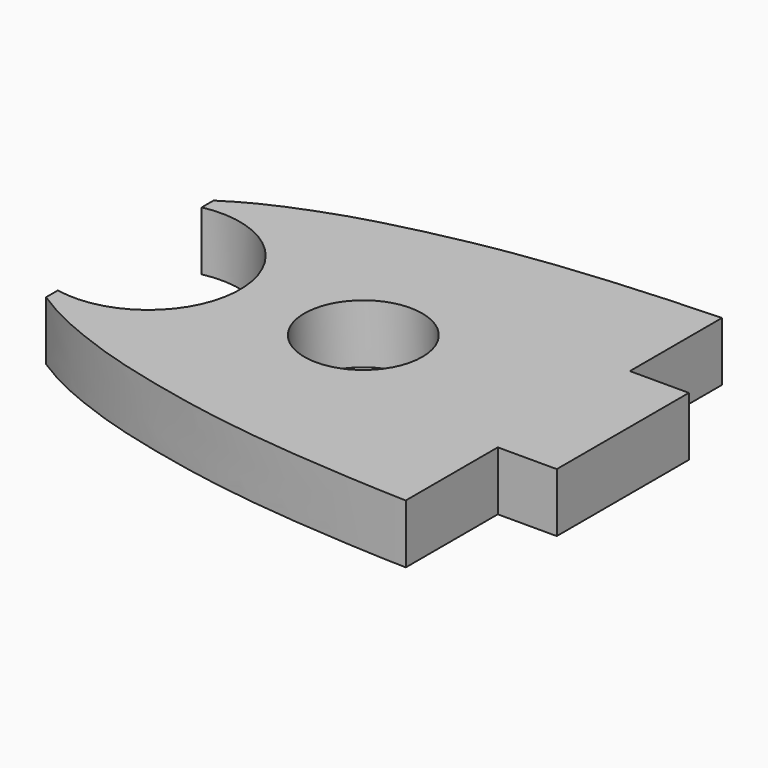
from build123d import *

# Parameters (mm, degrees)
F1_DEPTH      = 3.175
F2_R          = 3.175
F3_DEPTH      = 3.175
F4_W          = 1.27
F4_H          = 6.2519614453
F5_DEPTH      = 25.4
F5_DEPTH_BACK = 25.4


with BuildPart() as f1:
    # F0 (on Top) → F1 (new body)
    with BuildSketch(Plane.XY):
        with BuildLine():
            Line((27.305, 4.445), (27.305, 10.639110318))
            add(Edge.make_bspline(
                [(27.305, 10.639110318), (26.6654543063, 10.6206147569), (24.478766488, 10.5308275824), (20.2410001582, 10.2440182138), (15.3587302448, 9.6192519425), (10.1940451056, 8.4075577542), (7.6509138704, 7.5021601175), (5.5897078561, 6.6511520763), (4.3073818225, 5.8741162544), (3.9357558202, 5.633461687)],
                knots=[0.3056468503, 0.3056468503, 0.3056468503, 0.3056468503, 0.3165359722, 0.343963226, 0.3714836424, 0.3992368185, 0.4191371497, 0.4394264313, 0.4482604373, 0.4482604373, 0.4482604373, 0.4482604373], degree=3))
            Line((3.9357558202, 5.633461687), (3.9357558202, 4.839711687))
            ThreePointArc((3.9357558202, 4.839711687), (9.8679, 0), (3.9357558202, -4.839711687))
            Line((3.9357558202, -4.839711687), (3.9357558202, -5.633461687))
            add(Edge.make_bspline(
                [(3.9357558202, -5.633461687), (4.3073818225, -5.8741162544), (5.5897078561, -6.6511520763), (7.6509138704, -7.5021601175), (10.1940451056, -8.4075577542), (15.3587302448, -9.6192519425), (20.2410001582, -10.2440182138), (24.478766488, -10.5308275824), (26.6654543063, -10.6206147569), (27.305, -10.639110318)],
                knots=[0.5517395627, 0.5517395627, 0.5517395627, 0.5517395627, 0.5605735687, 0.5808628503, 0.6007631815, 0.6285163576, 0.656036774, 0.6834640278, 0.6943531497, 0.6943531497, 0.6943531497, 0.6943531497], degree=3))
            Line((27.305, -10.639110318), (27.305, -4.445))
            Line((27.305, -4.445), (30.48, -4.445))
            Line((30.48, -4.445), (30.48, 4.445))
            Line((30.48, 4.445), (27.305, 4.445))
        make_face()
    extrude(amount=F1_DEPTH)

    # F2 (on face) → F3 (cut, through all)
    with BuildSketch(Plane.XY.offset(3.175)):
        with Locations((16.51, 0)):
            Circle(F2_R)
    extrude(amount=-F3_DEPTH, mode=Mode.SUBTRACT)


with BuildPart() as f1b:
    # F0 (on Top) → F1, piece 2 (new body)
    with BuildSketch(Plane.XY):
        with BuildLine():
            add(Edge.make_bspline(
                [(1.1020531618, 3.1259807227), (0.5678867915, 2.3248543379), (-0.5678867915, 0), (0.5678867915, -2.3248543379), (1.1020531618, -3.1259807227)],
                knots=[0.4791511417, 0.4791511417, 0.4791511417, 0.4791511417, 0.5, 0.5208488583, 0.5208488583, 0.5208488583, 0.5208488583], degree=3))
            ThreePointArc((1.1020531618, 3.1259807227), (-0.0127, 0), (1.1020531618, -3.1259807227))
        make_face()
    extrude(amount=F1_DEPTH)

    # F4 (on Top) → F5 (cut, two sides)
    with BuildSketch(Plane.XY) as f5_sk:
        with Locations((0.4670531618, 0)):
            Rectangle(F4_W, F4_H)
    extrude(amount=F5_DEPTH, mode=Mode.SUBTRACT)
    extrude(f5_sk.sketch, amount=-F5_DEPTH_BACK, mode=Mode.SUBTRACT)


solid = f1.part
